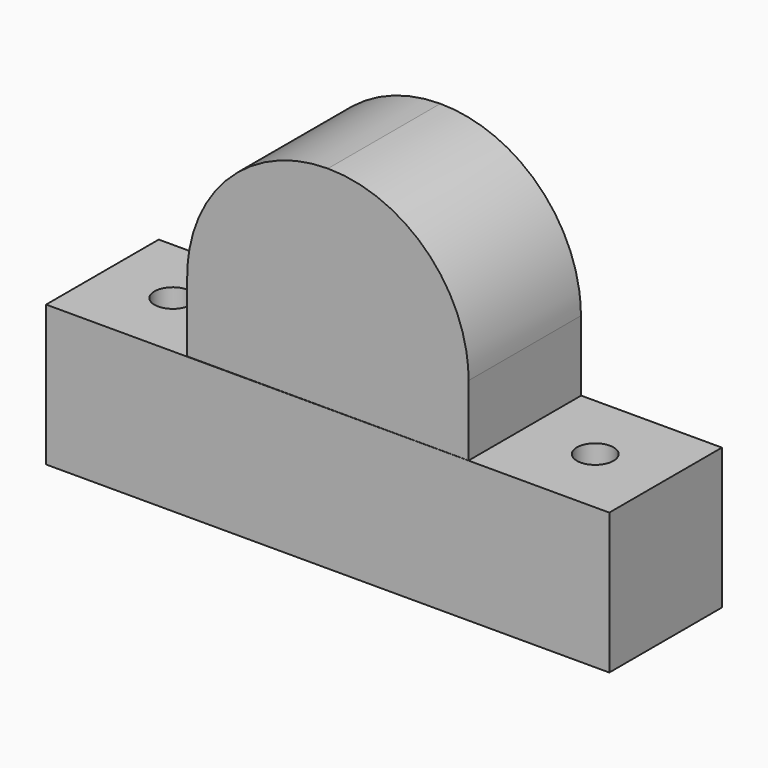
from build123d import *

# Parameters (mm, degrees)
F2_DEPTH = 31.75
F0_W     = 50.8
F0_H     = 12.7
F0_R     = 1.651
F3_DEPTH = 12.7
F4_R     = 12.7
F5_R     = 12.69999


# Not quite as in the source:
# - a fillet or chamfer is up to 0.001 mm smaller than in the source, because OpenCascade refuses the exact size


with BuildPart() as f2:
    # F1 (on face) → F2 (new body)
    with BuildSketch(Plane.XY):
        Polygon((12.7, -6.3331015408), (12.7, 6.3278423622), (7.1869615835, 6.35), (-12.7, 6.35), (-12.7, -6.310286466), align=None)
    extrude(amount=F2_DEPTH)

    # F0 (on Top) → F3 (join)
    with BuildSketch(Plane.XY):
        Rectangle(F0_W, F0_H)
        with Locations((-19.05, 0)):
            Circle(F0_R, mode=Mode.SUBTRACT)
        with Locations((19.05, 0)):
            Circle(F0_R, mode=Mode.SUBTRACT)
    extrude(amount=F3_DEPTH)

    # F4
    f4_edges = [f2.edges().sort_by_distance(p)[0] for p in [
        (-12.7, 0.019857, 31.75),
    ]]
    fillet(f4_edges, radius=F4_R)

    # F5 (radius 12.7 in the source; OpenCascade refuses exactly that, so slightly less here)
    f5_edges = [f2.edges().sort_by_distance(p)[0] for p in [
        (12.7, -0.00263, 31.75),
    ]]
    fillet(f5_edges, radius=F5_R)


solid = f2.part
